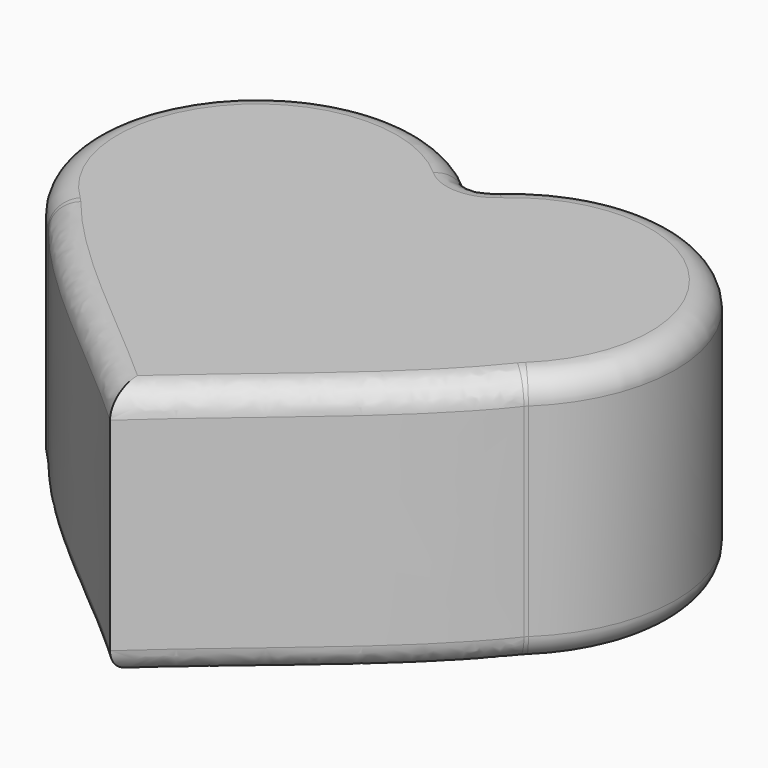
from build123d import *

# Parameters (mm, degrees)
F1_DEPTH = 10
F2_F1_R  = 1
F2_F2_R  = 1


with BuildPart() as f1:
    # F0 (on Top) → F1 (new body)
    with BuildSketch(Plane.XY):
        with BuildLine():
            ThreePointArc((9.4193928047, -1.2664417795), (9.4693151315, 8.2196633625), (0, 7.6533119315))
            ThreePointArc((0, 7.6533119315), (-9.4693151315, 8.2196633625), (-9.4193928047, -1.2664417795))
            add(Edge.make_bspline(
                [(0, -10), (-3.1397976016, -7.0888139265), (-6.9542042911, -4.3797008693), (-9.4193928047, -1.2664417795)],
                knots=[0, 0, 0, 0, 12.8452325787, 12.8452325787, 12.8452325787, 12.8452325787], degree=3))
            add(Edge.make_bspline(
                [(0, -10), (3.1397976016, -7.0888139265), (6.9542042911, -4.3797008693), (9.4193928047, -1.2664417795)],
                knots=[0, 0, 0, 0, 12.8452325787, 12.8452325787, 12.8452325787, 12.8452325787], degree=3))
        make_face()
    extrude(amount=F1_DEPTH)

    # F2: fillet of radius 1 on 7 edges, made by hand

    # F2_f1
    f2_f1_edges = [f1.edges().sort_by_distance(p)[0] for p in [
        (0, 7.6533119315, 5),
        (-9.4193928047, -1.2664417795, 5),
        (9.4193928047, -1.2664417795, 5),
    ]]
    fillet(f2_f1_edges, radius=F2_F1_R)

    # F2_f2
    f2_f2_edges = [f1.edges().sort_by_distance(p)[0] for p in [
        (-9.7828337858, 7.9016475299, 0),
        (-9.7828337858, 7.9016475299, 10),
        (9.7828337858, 7.9016475299, 0),
        (9.7828337858, 7.9016475299, 10),
        (9.4202986519, -1.2694012696, 10),
        (1e-10, 8.0901699416, 10),
        (9.4202986519, -1.2694012696, 0),
        (1e-10, 8.0901699416, 0),
        (-9.4202986519, -1.2694012696, 10),
        (-9.4202986519, -1.2694012696, 0),
    ]]
    fillet(f2_f2_edges, radius=F2_F2_R)


solid = f1.part
